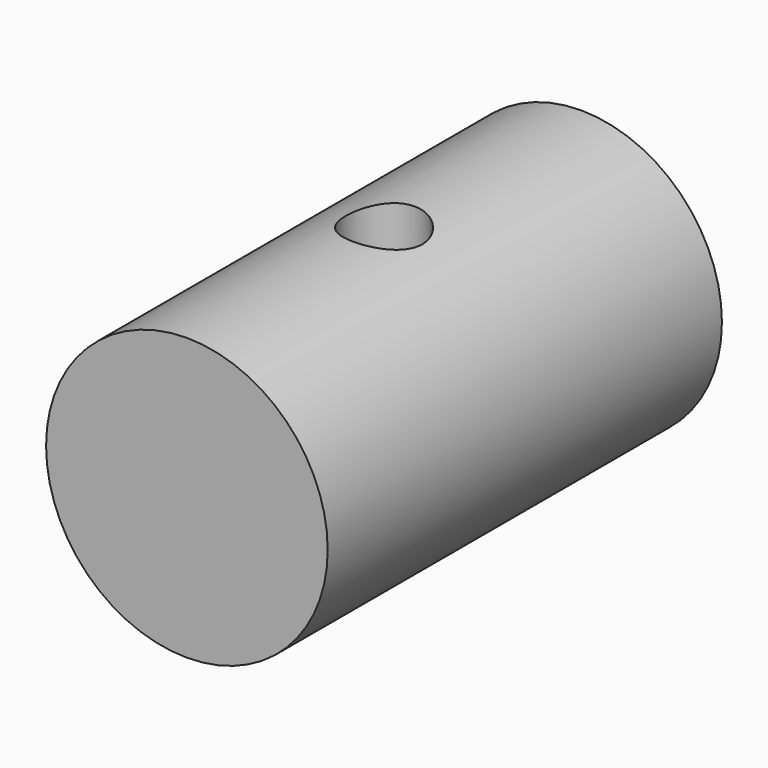
from build123d import *

# Parameters (mm, degrees)
F0_R     = 6.35
F1_DEPTH = 11.1125
F3_D     = 3.4544
F3_DEPTH = 9.525
F3_TIP   = 1.0378064612


with BuildPart() as f1:
    # F0 (on Front) → F1 (new body, symmetric)
    with BuildSketch(Plane.XZ):
        with Locations((0, -6.35)):
            Circle(F0_R)
    extrude(amount=F1_DEPTH, both=True)

    # F3 (one way)
    with BuildSketch(Plane.XY):
        with Locations((0, 0)):
            Circle(F3_D / 2)
    extrude(amount=-F3_DEPTH, mode=Mode.SUBTRACT)
    with Locations(Plane.XY):
        with Locations((0, 0)):
            with Locations((0, 0, -(F3_DEPTH + F3_TIP / 2))):  # 118° drill point
                Cone(0, F3_D / 2, F3_TIP, mode=Mode.SUBTRACT)


solid = f1.part
